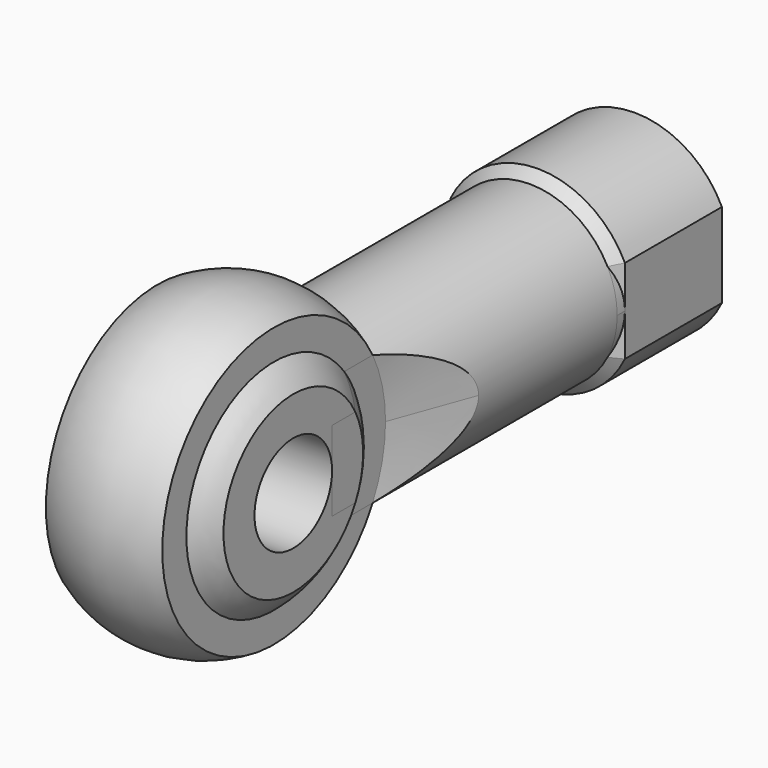
from build123d import *

# Parameters (mm, degrees)
F9_R          = 2.5
F10_DEPTH     = 24.5
F11_DEPTH     = 6.75
F12_DEPTH     = 14
F13_T2_ANGLE  = 157.8095212227
F13_T6_DEPTH  = 3.4652909658
F13_S7_R      = 4.5
F13_T8_DEPTH  = 3
F13_T12_DEPTH = 3.4652909658
F13_S13_R     = 4.5
F13_T14_DEPTH = 3
F13_T16_ANGLE = 157.8095212227
F13_T20_DEPTH = 3.4652909658
F13_S21_R     = 4.5
F13_T22_DEPTH = 3
F13_T26_DEPTH = 3.4652909658
F13_S27_R     = 4.5
F13_T28_DEPTH = 3


# Not quite as in the source:
# - a fillet or chamfer that OpenCascade refuses, or shapes differently, is made with other operations: its cross-section is extruded or revolved along the edge and cut away or added


with BuildPart() as f7:
    # F6 (on Top) → F7 (revolve)
    with BuildSketch(Plane.XY):
        with BuildLine():
            Line((-4, 4.5), (-4, 2.5))
            Line((-4, 2.5), (4, 2.5))
            Line((4, 2.5), (4, 4.5))
            ThreePointArc((4, 4.5), (3.5461149614, 5.1104772433), (3, 5.6400549446))
            ThreePointArc((3, 5.6400549446), (0, 6.716990566), (-3, 5.6400549446))
            ThreePointArc((-3, 5.6400549446), (-3.5461149614, 5.1104772433), (-4, 4.5))
        make_face()
        with BuildLine():
            Line((-3, 7.1961524227), (-3, 5.6400549446))
            ThreePointArc((-3, 5.6400549446), (0, 6.716990566), (3, 5.6400549446))
            Line((3, 5.6400549446), (3, 7.1961524227))
            ThreePointArc((3, 7.1961524227), (0, 8), (-3, 7.1961524227))
        make_face()
    revolve(axis=Axis((0, 0, 0), (1, 0, 0)))

    # F9 (on offset) → F10 (join)
    with BuildSketch(Plane.XZ.offset(-27)):
        with BuildLine():
            ThreePointArc((-4.5, 0), (0, -4.5), (4.5, 0))
            ThreePointArc((4.5, 0), (0, 4.5), (-4.5, 0))
        make_face()
        Circle(F9_R, mode=Mode.SUBTRACT)
        Circle(F9_R)
    extrude(amount=F10_DEPTH)

    # F9 (on offset) → F11 (join)
    with BuildSketch(Plane.XZ.offset(-27)):
        with BuildLine():
            ThreePointArc((-4.5, 0), (0, 4.5), (4.5, 0))
            Line((4.5, 0), (4.5, 2.1794494718))
            ThreePointArc((4.5, 2.1794494718), (0, 5), (-4.5, 2.1794494718))
            Line((-4.5, 2.1794494718), (-4.5, 0))
        make_face()
        with BuildLine():
            Line((4.5, -2.1794494718), (4.5, 0))
            ThreePointArc((4.5, 0), (0, -4.5), (-4.5, 0))
            Line((-4.5, 0), (-4.5, -2.1794494718))
            ThreePointArc((-4.5, -2.1794494718), (0, -5), (4.5, -2.1794494718))
        make_face()
    extrude(amount=F11_DEPTH)

    # F9 (on offset) → F12 (cut)
    with BuildSketch(Plane.XZ.offset(-27)):
        Circle(F9_R)
    extrude(amount=F12_DEPTH, mode=Mode.SUBTRACT)

    # F13: chamfer of 0.5 on 6 edges, made by hand

    # F13_s1 → F13_t2 (revolve, cut)
    with BuildSketch(Plane(origin=(0, 0, 0), x_dir=(0, 1, 0), z_dir=(0.1924404319, 0, -0.9813086569))):
        Polygon((20.25, 4.5), (20.75, 5), (20.25, 5), align=None)
    revolve(axis=Axis((0, 20.25, 0), (0, -1, 0)), revolution_arc=F13_T2_ANGLE, mode=Mode.SUBTRACT)


with BuildPart() as f13_tool4:
    # F13_s5 → F13_t6 (new body)
    with BuildSketch(Plane.XY):
        Polygon((4, 20.25), (4.5, 20.75), (4.5, 20.25), align=None)
    extrude(amount=F13_T6_DEPTH)

    # F13_s7 → F13_t8 (cut, symmetric)
    with BuildSketch(Plane.XZ.offset(-20.5)):
        Circle(F13_S7_R)
    extrude(amount=F13_T8_DEPTH, both=True, mode=Mode.SUBTRACT)


with BuildPart() as f7_1:
    add(f7.part)

    # F13_t3: cut F13_tool4
    add(f13_tool4.part, mode=Mode.SUBTRACT)


with BuildPart() as f13_tool10:
    # F13_s11 → F13_t12 (new body)
    with BuildSketch(Plane.XY.offset(3.4652909658)):
        Polygon((-4, 20.25), (-4.5, 20.75), (-4.5, 20.25), align=None)
    extrude(amount=-F13_T12_DEPTH)

    # F13_s13 → F13_t14 (cut, symmetric)
    with BuildSketch(Plane.XZ.offset(-20.5)):
        Circle(F13_S13_R)
    extrude(amount=F13_T14_DEPTH, both=True, mode=Mode.SUBTRACT)


with BuildPart() as f7_2:
    add(f7_1.part)

    # F13_t9: cut F13_tool10
    add(f13_tool10.part, mode=Mode.SUBTRACT)

    # F13_s15 → F13_t16 (revolve, cut)
    with BuildSketch(Plane(origin=(0, 0, 0), x_dir=(0, 1, 0), z_dir=(-0.1924404319, 0, 0.9813086569))):
        Polygon((20.25, 4.5), (20.75, 5), (20.25, 5), align=None)
    revolve(axis=Axis((0, 20.25, 0), (0, -1, 0)), revolution_arc=F13_T16_ANGLE, mode=Mode.SUBTRACT)


with BuildPart() as f13_tool18:
    # F13_s19 → F13_t20 (new body)
    with BuildSketch(Plane.XY.offset(-3.4652909658)):
        Polygon((4, 20.25), (4.5, 20.75), (4.5, 20.25), align=None)
    extrude(amount=F13_T20_DEPTH)

    # F13_s21 → F13_t22 (cut, symmetric)
    with BuildSketch(Plane.XZ.offset(-20.5)):
        Circle(F13_S21_R)
    extrude(amount=F13_T22_DEPTH, both=True, mode=Mode.SUBTRACT)


with BuildPart() as f7_3:
    add(f7_2.part)

    # F13_t17: cut F13_tool18
    add(f13_tool18.part, mode=Mode.SUBTRACT)


with BuildPart() as f13_tool24:
    # F13_s25 → F13_t26 (new body)
    with BuildSketch(Plane.XY):
        Polygon((-4, 20.25), (-4.5, 20.75), (-4.5, 20.25), align=None)
    extrude(amount=-F13_T26_DEPTH)

    # F13_s27 → F13_t28 (cut, symmetric)
    with BuildSketch(Plane.XZ.offset(-20.5)):
        Circle(F13_S27_R)
    extrude(amount=F13_T28_DEPTH, both=True, mode=Mode.SUBTRACT)


with BuildPart() as f7_4:
    add(f7_3.part)

    # F13_t23: cut F13_tool24
    add(f13_tool24.part, mode=Mode.SUBTRACT)

    # F6 (on Top) → F14 (revolve, cut)
    with BuildSketch(Plane.XY):
        with BuildLine():
            Line((4, 4.5), (4, 2.5))
            Line((4, 2.5), (6, 2.5))
            Line((6, 2.5), (6, 15.4385846811))
            Line((6, 15.4385846811), (3, 7.1961524227))
            Line((3, 7.1961524227), (3, 5.6400549446))
            ThreePointArc((3, 5.6400549446), (3.5461149614, 5.1104772433), (4, 4.5))
        make_face()
        with BuildLine():
            Line((-6, 2.5), (-4, 2.5))
            Line((-4, 2.5), (-4, 4.5))
            ThreePointArc((-4, 4.5), (-3.5461149614, 5.1104772433), (-3, 5.6400549446))
            Line((-3, 5.6400549446), (-3, 7.1961524227))
            Line((-3, 7.1961524227), (-6, 15.4385846811))
            Line((-6, 15.4385846811), (-6, 2.5))
        make_face()
    revolve(axis=Axis((0, 0, 0), (1, 0, 0)), mode=Mode.SUBTRACT)


solid = f7_4.part
